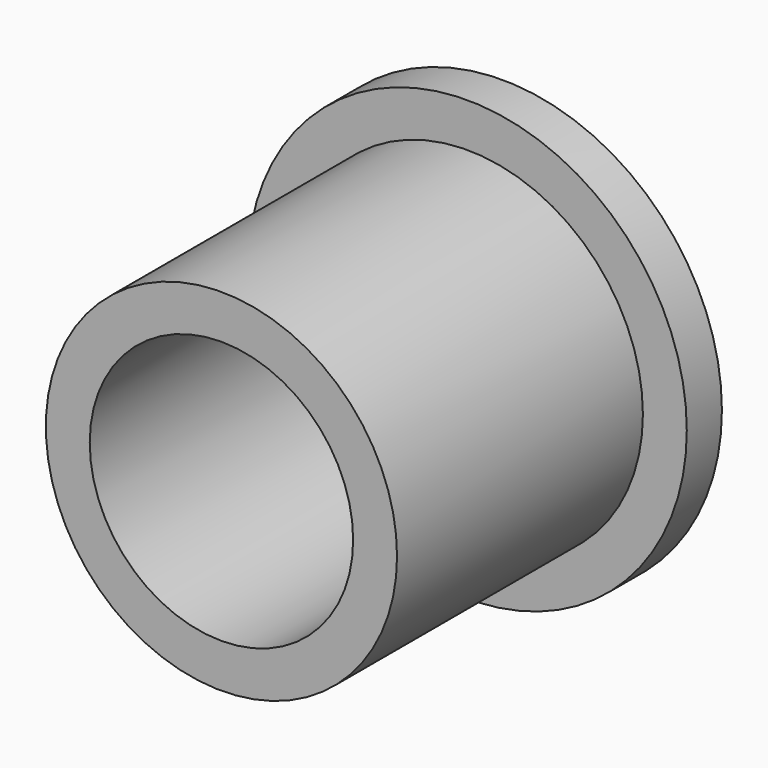
from build123d import *

# Parameters (mm, degrees)
F0_R     = 15.875
F0_R_2   = 12.7
F0_R_3   = 9.525
F1_DEPTH = 3.175
F3_DEPTH = 22.225


# Not quite as in the source:
# - a feature of the source that left no trace in its solid (it failed there, or was rolled back) is left out


with BuildPart() as f1:
    # F0 (on Front) → F1 (new body)
    with BuildSketch(Plane.XZ):
        Circle(F0_R)
        Circle(F0_R_2, mode=Mode.SUBTRACT)
        Circle(F0_R_2)
        Circle(F0_R_3, mode=Mode.SUBTRACT)
    extrude(amount=-F1_DEPTH)

    # F0 (on Front) → F3 (join)
    with BuildSketch(Plane.XZ):
        Circle(F0_R_2)
        Circle(F0_R_3, mode=Mode.SUBTRACT)
    extrude(amount=F3_DEPTH)


solid = f1.part
